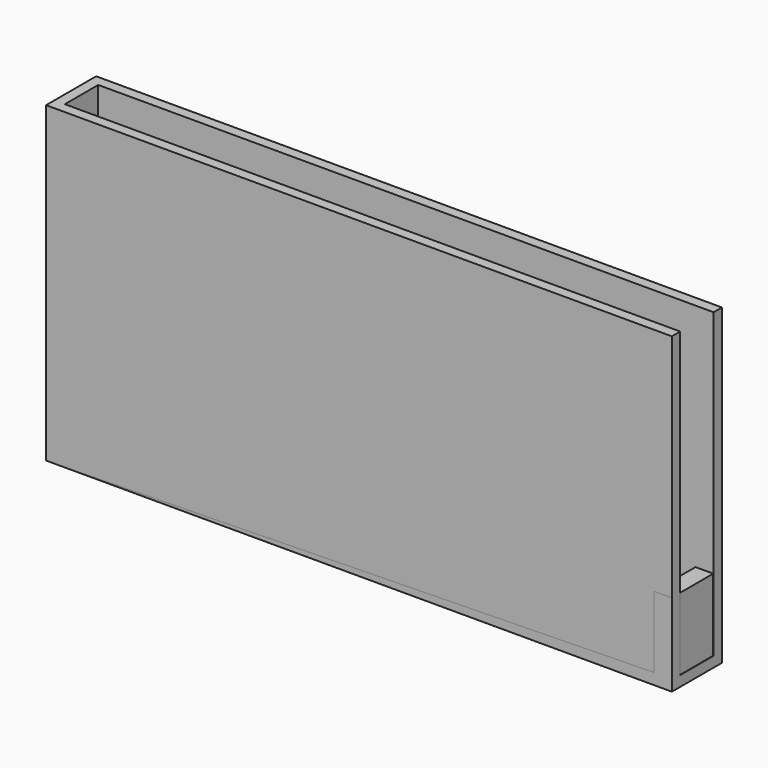
from build123d import *

# Parameters (mm, degrees)
F0_W     = 150
F0_H     = 75
F1_DEPTH = 15
F2_T     = -2.5
F4_DEPTH = 15
F5_W     = 4.2480379343
F5_H     = 19.8161639273
F6_DEPTH = 15


with BuildPart() as f1:
    # F0 (on Front) → F1 (new body)
    with BuildSketch(Plane.XZ):
        with Locations((75, 37.5)):
            Rectangle(F0_W, F0_H)
    extrude(amount=F1_DEPTH)

    # F2
    f2_openings = [f1.faces().sort_by_distance(p)[0] for p in [
        (75, -7.5, 75),
        (150, -7.5, 37.5),
    ]]
    offset(amount=F2_T, openings=f2_openings)


with BuildPart() as f4:
    # F3 (on Front) → F4 (new body)
    with BuildSketch(Plane.XZ):
        Polygon((149.8608291149, 2.7603094932), (0, 0), (149.9116716769, 0), align=None)
    extrude(amount=F4_DEPTH)

    # F5 (on face) → F6 (join)
    with BuildSketch(Plane.XZ):
        with Locations((147.7968916297, 9.9080819637)):
            Rectangle(F5_W, F5_H)
    extrude(amount=F6_DEPTH)


solid = Compound([f1.part, f4.part])
